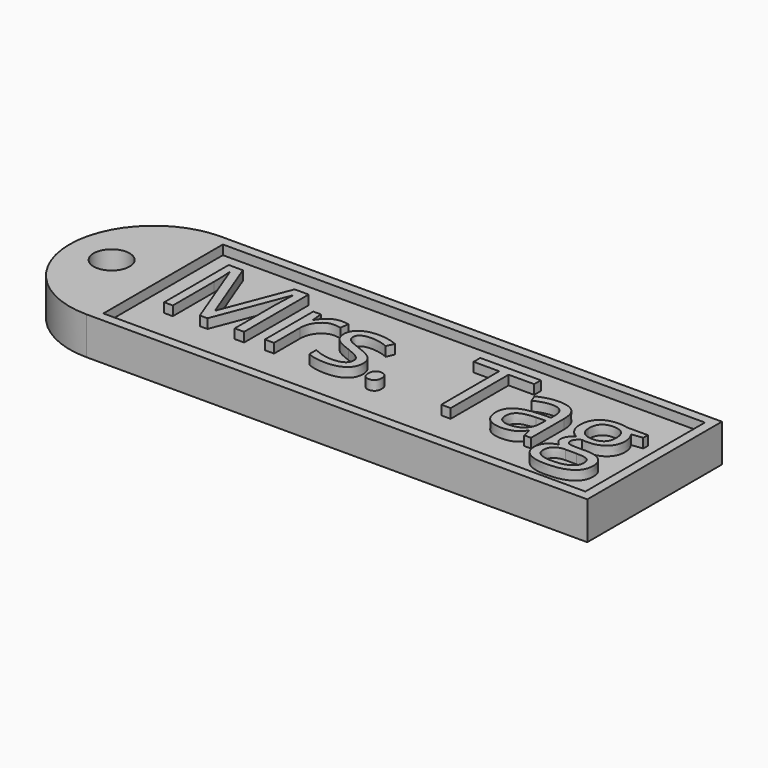
from build123d import *

# Parameters (mm, degrees)
F0_R         = 1.905
F1_DEPTH     = 4
F2_W         = 51.067
F2_H         = 15.828
F3_DEPTH     = 1
F4_TEXT_SIZE = 11.9802476828
F5_DEPTH     = 1


# Not quite as in the source:
# - Text() gives the source's letters only with a copy of the font that has no kerning and outlines rounded to 1/6400 em; it was checked with that copy


with BuildPart() as f1:
    # F0 (on Top) → F1 (new body)
    with BuildSketch(Plane.XY):
        with BuildLine():
            ThreePointArc((0, 17.828), (-8.914, 8.914), (0, 0))
            Line((0, 0), (53.067, 0))
            Line((53.067, 0), (53.067, 17.828))
            Line((53.067, 17.828), (0, 17.828))
        make_face()
        with Locations((-4.457, 8.914)):
            Circle(F0_R, mode=Mode.SUBTRACT)
    extrude(amount=F1_DEPTH)

    # F2 (on face) → F3 (cut)
    with BuildSketch(Plane.XY.offset(4)):
        with Locations((26.5335, 8.914)):
            Rectangle(F2_W, F2_H)
    extrude(amount=-F3_DEPTH, mode=Mode.SUBTRACT)

    # F4 (on face) → F5 (join)
    with BuildSketch(Plane.XY.offset(3)):
        with Locations((2.5, 5.7022216684)):
            Text('Mrs. Tag', F4_TEXT_SIZE, font='Open Sans', text_align=(TextAlign.LEFT, TextAlign.BOTTOM))
    extrude(amount=F5_DEPTH)


solid = f1.part
